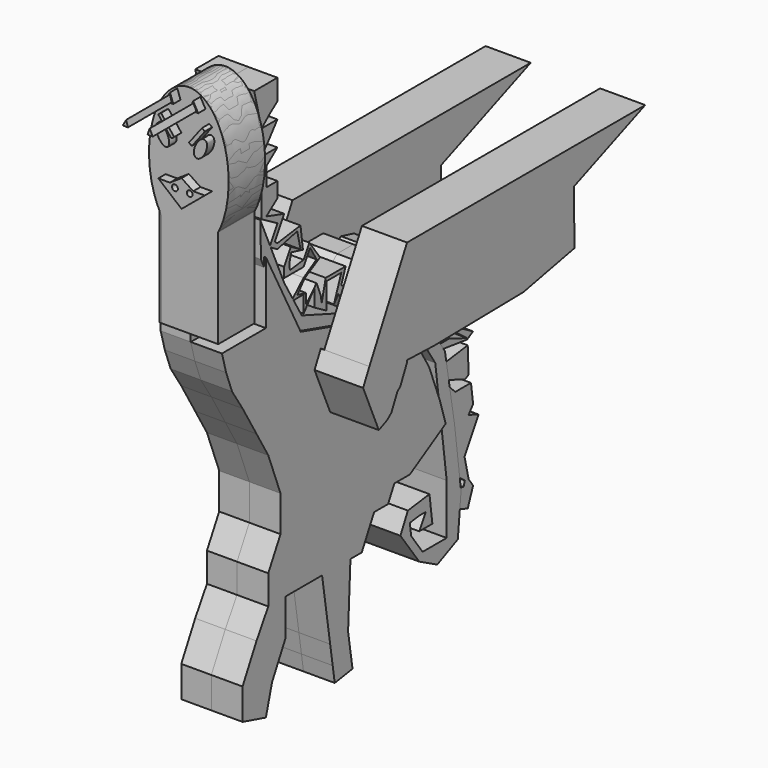
from build123d import *

# Parameters (mm, degrees)
F2_DEPTH        = 10
F3_DEPTH        = 12
F6_DEPTH        = 12
F9_DEPTH        = 6.4516
F10_DEPTH       = 6.858
F12_DEPTH       = 6.858
F11_W           = 12.0658394881
F11_H           = 1.8816260854
F13_DEPTH       = 6.604
F15_DEPTH       = 17.526
F17_DEPTH       = 9.906
F7_R            = 0.6318129406
F19_DEPTH       = 2
F20_R           = 0.6513123698
F21_DEPTH       = 2
F23_DEPTH       = 6.35
F24_DEPTH       = 6.604
F25_T1_DEPTH    = 30.4879557141
F25_T6_DEPTH    = 38.0832620454
F25_T11_DEPTH   = 30.8249260125
F25_2_T1_DEPTH  = 30.4879557141
F25_2_T6_DEPTH  = 38.0832620454
F25_2_T11_DEPTH = 30.8249260125
F27_DEPTH       = 2


# Not quite as in the source:
# - a fillet or chamfer that OpenCascade refuses, or shapes differently, is made with other operations: its cross-section is extruded or revolved along the edge and cut away or added


with BuildPart() as f2:
    # F0 (on Front) → F2 (new body)
    with BuildSketch(Plane.XZ):
        with BuildLine():
            add(Edge.make_bspline(
                [(-6.4547309206, 21.6429212113), (-3.8551533155, 16.5975436478), (0, 16.5975436478)],
                knots=[5.452422114, 5.452422114, 5.452422114, 6.2831853072, 6.2831853072, 6.2831853072], degree=2, weights=[1, 0.914962398, 1]))
            add(Edge.make_bspline(
                [(0, 16.5975436478), (3.434445083, 16.5975436478), (5.9502786025, 20.7410475478)],
                knots=[0, 0, 0, 0.7487654274, 0.7487654274, 0.7487654274], degree=2, weights=[1, 0.9307335396, 1]))
            add(Edge.make_bspline(
                [(5.9502786025, 20.7410475478), (21.313577746, 46.0439499156), (0.3582693213, 47.5674506226), (-20.5970391034, 49.0909513296), (-6.4547309206, 21.6429212113)],
                knots=[0.7487654274, 0.7487654274, 0.7487654274, 3.1005937707, 3.1005937707, 5.452422114, 5.452422114, 5.452422114], degree=2, weights=[1, 0.3846994157, 1, 0.3846994157, 1]))
        make_face()
        with BuildLine():
            add(Edge.make_bspline(
                [(0, 16.5975436478), (3.434445083, 16.5975436478), (5.9502786025, 20.7410475478)],
                knots=[0, 0, 0, 0.7487654274, 0.7487654274, 0.7487654274], degree=2, weights=[1, 0.9307335396, 1]))
            add(Edge.make_bspline(
                [(-6.4547309206, 21.6429212113), (-3.8551533155, 16.5975436478), (0, 16.5975436478)],
                knots=[5.452422114, 5.452422114, 5.452422114, 6.2831853072, 6.2831853072, 6.2831853072], degree=2, weights=[1, 0.914962398, 1]))
            Line((-6.4547309206, 21.6429212113), (-6.4547309206, 0))
            Line((-6.4547309206, 0), (5.9502786025, 0))
            Line((5.9502786025, 0), (5.9502786025, 20.7410475478))
        make_face()
    extrude(amount=F2_DEPTH)

    # F26 (on face) → F27 (join)
    with BuildSketch(Plane.XZ.offset(10)):
        with BuildLine():
            add(Edge.make_bspline(
                [(-3.1401312444, 35.7701145113), (-1.3681655429, 36.6560967536), (-3.7799722355, 39.2647554115), (-6.191778928, 41.8734140694), (-5.551937937, 38.3787731691), (-4.912096946, 34.8841322689), (-3.1401312444, 35.7701145113)],
                knots=[0, 0, 0, 2.0943951024, 2.0943951024, 4.1887902048, 4.1887902048, 6.2831853072, 6.2831853072, 6.2831853072], degree=2, weights=[1, 0.5, 1, 0.5, 1, 0.5, 1]))
        make_face()
    extrude(amount=F27_DEPTH)


with BuildPart() as f3:
    # F1 (on Front) → F3 (new body)
    with BuildSketch(Plane.XZ):
        Polygon((0, 29.1138663888), (0, 30.8139454573), (-2.5501206983, 29.1138663888), (-5.1002390683, 29.1138663888), (0, 24.8636659235), align=None)
    extrude(amount=F3_DEPTH)

    # F4: F3, F3b, F3c across plane


with BuildPart() as f3b:
    # F1 (on Front) → F3, piece 2 (new body)
    with BuildSketch(Plane.XZ):
        Polygon((-4.9794949527, 41.5934874921), (-5.0889090635, 41.4394438267), (-2.3262791801, 37.8267727792), (-2.0990670114, 37.8267727792), align=None)
        Polygon((-4.4865803793, 41.9569909573), (-4.9794949527, 41.5934874921), (-2.0990670114, 37.8267727792), (-1.6342759562, 38.227053165), align=None)
    extrude(amount=F3_DEPTH)


with BuildPart() as f3c:
    # F1 (on Front) → F3, piece 3 (new body)
    with BuildSketch(Plane.XZ):
        Polygon((-1.8204356311, 44.5381850004), (-2.5387881324, 46.5396828949), (-3.6612094846, 44.5381850004), align=None)
    extrude(amount=F3_DEPTH)


with BuildPart() as f3_1:
    add(f3.part)
    add(f3.part.mirror(Plane.YZ))
    add(f3b.part.mirror(Plane.YZ))
    add(f3c.part.mirror(Plane.YZ))

    # F7 (on face) → F19 (cut)
    with BuildSketch(Plane.XZ.offset(12)):
        with Locations((1.7824703828, 28.3940453082)):
            Circle(F7_R)
    extrude(amount=-F19_DEPTH, mode=Mode.SUBTRACT)

    # F20 (on face) → F21 (cut)
    with BuildSketch(Plane.XZ.offset(12)):
        with Locations((-1.4582620934, 28.475811705)):
            Circle(F20_R)
    extrude(amount=-F21_DEPTH, mode=Mode.SUBTRACT)


with BuildPart() as f6:
    # F5 (on face) → F6 (new body)
    with BuildSketch(Plane.XZ.offset(12)):
        Polygon((3.2756209839, 44.7876943326), (2.6005038526, 46.1258143187), (2.1202426234, 44.7876943326), align=None)
    extrude(amount=F6_DEPTH)


with BuildPart() as f6b:
    # F5 (on face) → F6, piece 2 (new body)
    with BuildSketch(Plane.XZ.offset(12)):
        Polygon((-2.162355464, 44.7876943326), (-2.5670824107, 46.1258143187), (-3.3061699942, 44.7876943326), align=None)
    extrude(amount=F6_DEPTH)


with BuildPart() as f9:
    # F8 (on Right) → F9 (new body)
    with BuildSketch(Plane.YZ):
        Polygon((8.1054354087, 4.4866758399), (1.532137394, 19.3184427917), (1.7557375602, 11.5948172129), (5.6305897209, 2.8517320687), (12.5971920788, -6.7422310822), (27.7625638992, -12.0216775686), (40.6580848693, -14.0168217382), (49.572861783, -27.8496284224), (51.4152313818, -41.9769918138), (52.6994355023, -51.8243201077), (52.6994355023, -62.9449018589), (46.0980413482, -62.9449018589), (42.9474816572, -58.6061507681), (42.596552131, -55.9152091975), (45.1674684882, -55.5799323304), (46.9695012919, -55.5799323304), (45.1674684882, -58.6061507681), (48.7715340956, -58.6061507681), (47.9822271747, -52.5537138927), (42.0558825135, -53.3265769482), (40.0054641068, -57.3544502258), (45.1674684882, -64.4632354379), (50.1269362867, -67.0540854335), (55.7603035122, -64.4632354379), (56.6465519369, -55.527344346), (54.8740550876, -41.9357679784), (52.2256828845, -26.6500413418), (42.817518115, -12.0516587049), (27.7625638992, -9.1861784458), (12.9205156118, -3.7682736292), align=None)
    extrude(amount=F9_DEPTH)

    # F8 (on Right) → F10 (join)
    with BuildSketch(Plane.YZ):
        Polygon((8.1054354087, 4.4866758399), (1.532137394, 19.3184427917), (1.7557375602, 11.5948172129), (5.6305897209, 2.8517320687), (12.5971920788, -6.7422310822), (27.7625638992, -12.0216775686), (40.6580848693, -14.0168217382), (49.572861783, -27.8496284224), (51.4152313818, -41.9769918138), (52.6994355023, -51.8243201077), (52.6994355023, -62.9449018589), (46.0980413482, -62.9449018589), (42.9474816572, -58.6061507681), (42.596552131, -55.9152091975), (45.1674684882, -55.5799323304), (46.9695012919, -55.5799323304), (45.1674684882, -58.6061507681), (48.7715340956, -58.6061507681), (47.9822271747, -52.5537138927), (42.0558825135, -53.3265769482), (40.0054641068, -57.3544502258), (45.1674684882, -64.4632354379), (50.1269362867, -67.0540854335), (55.7603035122, -64.4632354379), (56.6465519369, -55.527344346), (54.8740550876, -41.9357679784), (52.2256828845, -26.6500413418), (42.817518115, -12.0516587049), (27.7625638992, -9.1861784458), (12.9205156118, -3.7682736292), align=None)
    extrude(amount=-F10_DEPTH)

    # F11 (on Right) → F12 (join)
    with BuildSketch(Plane.YZ):
        Polygon((12.1393157169, -6.4757866785), (2.5822273456, 11.795071885), (2.5822273456, 0), (2.5822273456, -1.8816260854), (-9.4836121425, -1.8816260854), (-8.3336858079, -6.0433913022), (-6.721064914, -10.3481933475), (-3.8261981681, -14.8062761873), (0, -21.2691705674), (3.2231082692, -26.7133758606), (6.5893395804, -35.4489274323), (6.5893395804, -43.3371067047), (3.2231082692, -49.5215542614), (3.2231082692, -55.9407770634), (0, -61.2918324769), (-3.8261981681, -68.5529708862), (4.2684163239, -71.0125891538), (7.9679033037, -63.9919159361), (7.9679033037, -55.9407770634), (17.9930739105, -55.9407770634), (25.7815672235, -55.9407770634), (28.8898572326, -55.9407770634), (32.2724147794, -49.5215542614), (36.1035056412, -49.5215542614), (37.8392608134, -46.2275381138), (42.0941747725, -46.2275381138), (46.5768471874, -43.5736818115), (51.9265465413, -40.4065234666), (50.2568850148, -35.0830935564), (47.3863923786, -27.6340105488), (42.3810519278, -19.1794075072), (36.1895263195, -13.4464222938), align=None)
        Polygon((4.2684163239, -71.0125891538), (-3.8261981681, -68.5529708862), (-3.8261981681, -72.8864528992), (3.2231082692, -74.8211996529), align=None)
        Polygon((3.2231082692, -74.8211996529), (-3.8261981681, -72.8864528992), (-3.8261981681, -75.3974169493), (2.5822273456, -77.1562680602), align=None)
        Polygon((25.1365308756, -69.6748592245), (25.7815672235, -55.9407770634), (17.9930739105, -55.9407770634), (20.2164621664, -70.142770331), align=None)
        Polygon((25.7815672235, -73.795058135), (25.1365308756, -69.6748592245), (20.2164621664, -70.142770331), align=None)
        Polygon((25.7815672235, -73.795058135), (20.2164621664, -70.142770331), (20.9077002209, -74.5580847363), align=None)
        Polygon((26.3443690216, -77.3899801312), (25.7815672235, -73.795058135), (20.9077002209, -74.5580847363), (21.4705020189, -78.1530067325), align=None)
    extrude(amount=F12_DEPTH)

    # F22 (on Right) → F23 (join)
    with BuildSketch(Plane.YZ):
        Polygon((6.374317687, 21.5115565807), (2.0143464208, 19.2379765213), (6.374317687, 16.6825056076), (4.1873999871, 12.9513348546), (6.374317687, 11.6695363676), (11.8070757017, 12.9513348546), (12.7255132526, 9.0586410995), (10.064283419, 10.6184439099), (8.2402707776, 7.5064371706), (8.2402707776, 5.3265588358), (13.5636860505, 5.3265588358), (15.3341033033, 8.347124756), (17.1111002564, 5.3265588358), (13.5636860505, 3.2396173811), (10.1351579651, 0), (13.5636860505, 0), (13.5636860505, -3.7241033278), (16.5012590587, 0), (16.5012590587, -3.7241033278), (19.863597624, -5.6948407206), (19.863597624, 0), (23.9075515419, 0), (21.885574583, -5.2869431674), (23.1183427757, -3.7241033278), (25.1021422446, -7.5998823158), (30.3384047002, -2.1901051514), (34.0067259967, -2.1901051514), (30.6858606637, -5.7629146613), (30.6858606637, -9.3205478042), (38.5860130191, -4.9967369996), (42.6995791495, -4.9967369996), (40.7349355519, -7.5998823158), (36.7521606386, -8.9593110606), (36.7521606386, -11.3853020594), (41.0784259439, -14.0972314402), (43.5633193516, -7.5998823158), (48.0624114936, -9.3205478042), (48.0624114936, -11.3853020594), (44.4197580218, -12.4131189659), (43.1454405189, -14.9848153815), (52.4752251804, -14.9848153815), (54.5468328525, -18.7699061197), (49.4060702949, -16.8038355353), (45.3465212886, -19.0256562124), (48.0927578818, -24.0433798064), (51.1315829076, -22.3802087828), (54.3875972116, -23.6254625508), (58.4218000146, -26.6701526259), (53.4822099007, -24.7810198926), (48.0927578818, -24.7810198926), (50.4891980907, -29.1596209962), (50.9227966993, -29.1596209962), (50.4891980907, -25.9189717472), (58.4218000146, -26.9563752831), (60.0777398658, -26.0500673667), (56.1705380678, -23.7599741668), (55.147873642, -22.6992027075), (51.7546493685, -21.2227572942), (48.9587116034, -22.7529943547), (46.9672766634, -19.1143893965), (49.1664675286, -17.9107562517), (52.0101919188, -19.5775229623), (55.7815719124, -18.6877080364), (53.5723380744, -14.6511567863), (44.3100453781, -14.6511567863), (45.2610808354, -13.028564549), (48.8060855525, -12.1921603376), (50.4891980907, -9.3205478042), (43.5633193516, -6.3069887013), (41.0784259439, -10.5465454105), (37.872761488, -9.3205478042), (41.0784259439, -7.899916778), (43.5633193516, -4.6074424363), (40.0280356407, -3.7241033278), (31.8779945374, -7.5998823158), (32.7070372499, -5.2869431674), (35.1315699518, -1.1503698032), (30.6858606637, -1.1503698032), (26.6152015679, -4.9967369996), (23.9075515419, -2.3759328994), (25.1021422446, 0.7476106827), (19.6254998453, 0.7476106827), (18.5081807867, -3.7241033278), (18.3029319542, -2.1901051514), (17.1111002564, 0.7476106827), (14.2676095433, -2.1901051514), (14.2676095433, 0), (11.8434760085, 0.6057030017), (13.8522140785, 3.0138761345), (18.0777795613, 5.3265588358), (15.1306260624, 9.377462105), (13.5636860505, 6.7040552619), (9.805068531, 6.2011525404), (9.6304215526, 7.5064371706), (10.1351579651, 9.526484059), (13.3783222857, 8.7161349855), (12.7136140763, 13.6840618118), (6.374317687, 12.8358644653), (5.6650852585, 13.3711357547), (8.2402707776, 17.7647427445), (3.3210157141, 19.2379765213), align=None)
        Polygon((58.6017207746, -28.1321815733), (50.9227966993, -29.1596209962), (58.3676062524, -29.1596209962), (58.3676062524, -33.9571684599), (54.4010400298, -32.4401660534), (50.4891980907, -30.9440927994), (53.6639042409, -36.744684778), (58.487928737, -36.6766862571), (58.487928737, -40.385468403), (53.9383061336, -41.1653034389), (53.6639042409, -41.1653034389), (52.7907237411, -41.1653034389), (52.7907237411, -48.6471652985), (57.8177694986, -50.5697452036), (57.8177694986, -53.9344474673), (57.4758734829, -55.076067849), (57.8633627212, -55.192114329), (58.8622577488, -54.1251340254), (57.7316768195, -49.3332945378), (61.596813184, -42.7388608467), (58.8622577488, -41.6930375973), (60.0777398658, -40.0825284018), (59.4992414117, -35.7589200139), (55.147873642, -35.7589200139), (51.6759187848, -32.0609879557), (57.8940645443, -34.4391008), (58.8622577488, -33.909201622), align=None)
        Polygon((57.725328531, -48.586042255), (53.6639042409, -41.1653034389), (59.9615670733, -42.7388608467), align=None, mode=Mode.SUBTRACT)
        Polygon((50.9227966993, -29.1596209962), (50.4891980907, -29.1596209962), (50.4891980907, -30.9440927994), (54.4010400298, -32.4401660534), (58.3676062524, -33.9571684599), (58.3676062524, -29.1596209962), align=None)
        Polygon((57.2425117495, -55.8552828701), (57.4758734829, -55.076067849), (53.6639042409, -53.9344474673), (54.2127080262, -58.0361224711), (58.6017207746, -59.7146883964), (60.0777398658, -55.8552828701), (57.8633627212, -55.192114329), align=None)
        Polygon((59.9615670733, -42.7388608467), (53.6639042409, -41.1653034389), (57.725328531, -48.586042255), align=None)
        Polygon((3.3210157141, 24.8575396836), (2.0143464208, 24.8575396836), (2.0143464208, 19.2379765213), (6.374317687, 21.5115565807), (6.374317687, 24.8575396836), align=None)
        Polygon((57.8177694986, -50.5697452036), (52.7907237411, -48.6471652985), (53.6639042409, -50.7994458472), (57.8177694986, -53.9344474673), align=None)
        Polygon((58.487928737, -40.385468403), (53.6639042409, -36.744684778), (53.6639042409, -41.1653034389), (53.9383061336, -41.1653034389), align=None)
        Polygon((58.487928737, -36.6766862571), (53.6639042409, -36.744684778), (58.487928737, -40.385468403), align=None)
        Polygon((6.374317687, 31.3354618847), (2.0143464208, 31.3354618847), (2.0143464208, 27.9209110886), (3.3210157141, 28.9442409235), align=None)
        Polygon((3.3210157141, 28.9442409235), (2.0143464208, 27.9209110886), (2.0143464208, 24.8575396836), (3.3210157141, 24.8575396836), align=None)
        Polygon((58.8622577488, -54.1251340254), (57.8633627212, -55.192114329), (60.0777398658, -55.8552828701), align=None)
        Polygon((57.8633627212, -55.192114329), (57.4758734829, -55.076067849), (57.2425117495, -55.8552828701), align=None)
    extrude(amount=F23_DEPTH)


with BuildPart() as f13:
    # F11 (on Right) → F13 (new body)
    with BuildSketch(Plane.YZ):
        Polygon((12.1393157169, -6.4757866785), (2.5822273456, 11.795071885), (2.5822273456, 0), (2.5822273456, -1.8816260854), (-9.4836121425, -1.8816260854), (-8.3336858079, -6.0433913022), (-6.721064914, -10.3481933475), (-3.8261981681, -14.8062761873), (0, -21.2691705674), (3.2231082692, -26.7133758606), (6.5893395804, -35.4489274323), (6.5893395804, -43.3371067047), (3.2231082692, -49.5215542614), (3.2231082692, -55.9407770634), (0, -61.2918324769), (-3.8261981681, -68.5529708862), (4.2684163239, -71.0125891538), (7.9679033037, -63.9919159361), (7.9679033037, -55.9407770634), (17.9930739105, -55.9407770634), (25.7815672235, -55.9407770634), (28.8898572326, -55.9407770634), (32.2724147794, -49.5215542614), (36.1035056412, -49.5215542614), (37.8392608134, -46.2275381138), (42.0941747725, -46.2275381138), (46.5768471874, -43.5736818115), (51.9265465413, -40.4065234666), (50.2568850148, -35.0830935564), (47.3863923786, -27.6340105488), (42.3810519278, -19.1794075072), (36.1895263195, -13.4464222938), align=None)
        with Locations((-3.4506923985, -0.9408130427)):
            Rectangle(F11_W, F11_H)
        Polygon((25.1365308756, -69.6748592245), (25.7815672235, -55.9407770634), (17.9930739105, -55.9407770634), (20.2164621664, -70.142770331), align=None)
        Polygon((4.2684163239, -71.0125891538), (-3.8261981681, -68.5529708862), (-3.8261981681, -72.8864528992), (3.2231082692, -74.8211996529), align=None)
        Polygon((25.7815672235, -73.795058135), (25.1365308756, -69.6748592245), (20.2164621664, -70.142770331), align=None)
        Polygon((3.2231082692, -74.8211996529), (-3.8261981681, -72.8864528992), (-3.8261981681, -75.3974169493), (2.5822273456, -77.1562680602), align=None)
        Polygon((25.7815672235, -73.795058135), (20.2164621664, -70.142770331), (20.9077002209, -74.5580847363), align=None)
        Polygon((26.3443690216, -77.3899801312), (25.7815672235, -73.795058135), (20.9077002209, -74.5580847363), (21.4705020189, -78.1530067325), align=None)
    extrude(amount=-F13_DEPTH)


with BuildPart() as f15:
    # F14 (on Right) → F15 (new body)
    with BuildSketch(Plane.YZ):
        Polygon((17.6491290331, -11.953400448), (15.9272607416, -15.3971333057), (20.2319268137, -25.2978634089), (22.4355885149, -24.3397494456), (25.6127621979, -21.8541305512), (25.6127621979, -19.7017993778), (27.9803276062, -17.764698714), (27.9803276062, -14.7514333948), (25.6127621979, -14.7514333948), (22.4355885149, -14.7514333948), align=None)
    extrude(amount=F15_DEPTH)

    # F16 (on face) → F17 (join)
    with BuildSketch(Plane.YZ.offset(17.526)):
        Polygon((22.4355885149, -14.7514333948), (35.3657811751, -15.1493677909), (41.5879657357, -15.0487608429), (46.1636093004, -14.9747769342), (59.976618737, -14.7514333948), (73.9541649818, -11.953400448), (73.7608895935, 0), (93.3558419347, 7.8085386194), (27.9803276062, 7.8085386194), (17.6491290331, -11.953400448), align=None)
    extrude(amount=-F17_DEPTH)


with BuildPart() as f18_1:
    # F18: instance of F15
    add(f15.part.mirror(Plane.YZ))

    # F25#2: chamfer of 5.08 on 3 edges, made by hand

    # F25_2_s2 → F25_2_t1 (cut)
    with BuildSketch(Plane.YZ.offset(-24.0069778571)):
        Polygon((26.1171772651, -19.2890957802), (27.9803276062, -15.3573940784), (27.9803276062, -17.764698714), align=None)
    extrude(amount=F25_2_T1_DEPTH, mode=Mode.SUBTRACT)


with BuildPart() as f23:
    # F22 (on Right) → F23, piece 2 (new body)
    with BuildSketch(Plane.YZ):
        Polygon((6.374317687, 36.7647409439), (2.0143464208, 36.7647409439), (2.0143464208, 31.3354618847), (4.1873999871, 33.9406244457), align=None)
    extrude(amount=F23_DEPTH)


with BuildPart() as f23b:
    # F22 (on Right) → F23, piece 3 (new body)
    with BuildSketch(Plane.YZ):
        Polygon((6.374317687, 44.8229573667), (0, 44.8229573667), (2.0143464208, 36.7647409439), (4.1873999871, 38.6234745383), (6.374317687, 40.2723401785), (6.374317687, 42.8432300687), align=None)
    extrude(amount=F23_DEPTH)


with BuildPart() as f24:
    # F22 (on Right) → F24 (new body)
    with BuildSketch(Plane.YZ):
        Polygon((6.374317687, 21.5115565807), (2.0143464208, 19.2379765213), (6.374317687, 16.6825056076), (4.1873999871, 12.9513348546), (6.374317687, 11.6695363676), (11.8070757017, 12.9513348546), (12.7255132526, 9.0586410995), (10.064283419, 10.6184439099), (8.2402707776, 7.5064371706), (8.2402707776, 5.3265588358), (13.5636860505, 5.3265588358), (15.3341033033, 8.347124756), (17.1111002564, 5.3265588358), (13.5636860505, 3.2396173811), (10.1351579651, 0), (13.5636860505, 0), (13.5636860505, -3.7241033278), (16.5012590587, 0), (16.5012590587, -3.7241033278), (19.863597624, -5.6948407206), (19.863597624, 0), (23.9075515419, 0), (21.885574583, -5.2869431674), (23.1183427757, -3.7241033278), (25.1021422446, -7.5998823158), (30.3384047002, -2.1901051514), (34.0067259967, -2.1901051514), (30.6858606637, -5.7629146613), (30.6858606637, -9.3205478042), (38.5860130191, -4.9967369996), (42.6995791495, -4.9967369996), (40.7349355519, -7.5998823158), (36.7521606386, -8.9593110606), (36.7521606386, -11.3853020594), (41.0784259439, -14.0972314402), (43.5633193516, -7.5998823158), (48.0624114936, -9.3205478042), (48.0624114936, -11.3853020594), (44.4197580218, -12.4131189659), (43.1454405189, -14.9848153815), (52.4752251804, -14.9848153815), (54.5468328525, -18.7699061197), (49.4060702949, -16.8038355353), (45.3465212886, -19.0256562124), (48.0927578818, -24.0433798064), (51.1315829076, -22.3802087828), (54.3875972116, -23.6254625508), (58.4218000146, -26.6701526259), (53.4822099007, -24.7810198926), (48.0927578818, -24.7810198926), (50.4891980907, -29.1596209962), (50.9227966993, -29.1596209962), (50.4891980907, -25.9189717472), (58.4218000146, -26.9563752831), (60.0777398658, -26.0500673667), (56.1705380678, -23.7599741668), (55.147873642, -22.6992027075), (51.7546493685, -21.2227572942), (48.9587116034, -22.7529943547), (46.9672766634, -19.1143893965), (49.1664675286, -17.9107562517), (52.0101919188, -19.5775229623), (55.7815719124, -18.6877080364), (53.5723380744, -14.6511567863), (44.3100453781, -14.6511567863), (45.2610808354, -13.028564549), (48.8060855525, -12.1921603376), (50.4891980907, -9.3205478042), (43.5633193516, -6.3069887013), (41.0784259439, -10.5465454105), (37.872761488, -9.3205478042), (41.0784259439, -7.899916778), (43.5633193516, -4.6074424363), (40.0280356407, -3.7241033278), (31.8779945374, -7.5998823158), (32.7070372499, -5.2869431674), (35.1315699518, -1.1503698032), (30.6858606637, -1.1503698032), (26.6152015679, -4.9967369996), (23.9075515419, -2.3759328994), (25.1021422446, 0.7476106827), (19.6254998453, 0.7476106827), (18.5081807867, -3.7241033278), (18.3029319542, -2.1901051514), (17.1111002564, 0.7476106827), (14.2676095433, -2.1901051514), (14.2676095433, 0), (11.8434760085, 0.6057030017), (13.8522140785, 3.0138761345), (18.0777795613, 5.3265588358), (15.1306260624, 9.377462105), (13.5636860505, 6.7040552619), (9.805068531, 6.2011525404), (9.6304215526, 7.5064371706), (10.1351579651, 9.526484059), (13.3783222857, 8.7161349855), (12.7136140763, 13.6840618118), (6.374317687, 12.8358644653), (5.6650852585, 13.3711357547), (8.2402707776, 17.7647427445), (3.3210157141, 19.2379765213), align=None)
        Polygon((58.6017207746, -28.1321815733), (50.9227966993, -29.1596209962), (58.3676062524, -29.1596209962), (58.3676062524, -33.9571684599), (54.4010400298, -32.4401660534), (50.4891980907, -30.9440927994), (53.6639042409, -36.744684778), (58.487928737, -36.6766862571), (58.487928737, -40.385468403), (53.9383061336, -41.1653034389), (53.6639042409, -41.1653034389), (52.7907237411, -41.1653034389), (52.7907237411, -48.6471652985), (57.8177694986, -50.5697452036), (57.8177694986, -53.9344474673), (57.4758734829, -55.076067849), (57.8633627212, -55.192114329), (58.8622577488, -54.1251340254), (57.7316768195, -49.3332945378), (61.596813184, -42.7388608467), (58.8622577488, -41.6930375973), (60.0777398658, -40.0825284018), (59.4992414117, -35.7589200139), (55.147873642, -35.7589200139), (51.6759187848, -32.0609879557), (57.8940645443, -34.4391008), (58.8622577488, -33.909201622), align=None)
        Polygon((57.725328531, -48.586042255), (53.6639042409, -41.1653034389), (59.9615670733, -42.7388608467), align=None, mode=Mode.SUBTRACT)
        Polygon((50.9227966993, -29.1596209962), (50.4891980907, -29.1596209962), (50.4891980907, -30.9440927994), (54.4010400298, -32.4401660534), (58.3676062524, -33.9571684599), (58.3676062524, -29.1596209962), align=None)
        Polygon((57.2425117495, -55.8552828701), (57.4758734829, -55.076067849), (53.6639042409, -53.9344474673), (54.2127080262, -58.0361224711), (58.6017207746, -59.7146883964), (60.0777398658, -55.8552828701), (57.8633627212, -55.192114329), align=None)
        Polygon((59.9615670733, -42.7388608467), (53.6639042409, -41.1653034389), (57.725328531, -48.586042255), align=None)
        Polygon((3.3210157141, 24.8575396836), (2.0143464208, 24.8575396836), (2.0143464208, 19.2379765213), (6.374317687, 21.5115565807), (6.374317687, 24.8575396836), align=None)
        Polygon((57.8177694986, -50.5697452036), (52.7907237411, -48.6471652985), (53.6639042409, -50.7994458472), (57.8177694986, -53.9344474673), align=None)
        Polygon((58.487928737, -40.385468403), (53.6639042409, -36.744684778), (53.6639042409, -41.1653034389), (53.9383061336, -41.1653034389), align=None)
        Polygon((58.487928737, -36.6766862571), (53.6639042409, -36.744684778), (58.487928737, -40.385468403), align=None)
        Polygon((6.374317687, 31.3354618847), (2.0143464208, 31.3354618847), (2.0143464208, 27.9209110886), (3.3210157141, 28.9442409235), align=None)
        Polygon((3.3210157141, 28.9442409235), (2.0143464208, 27.9209110886), (2.0143464208, 24.8575396836), (3.3210157141, 24.8575396836), align=None)
        Polygon((58.8622577488, -54.1251340254), (57.8633627212, -55.192114329), (60.0777398658, -55.8552828701), align=None)
        Polygon((57.8633627212, -55.192114329), (57.4758734829, -55.076067849), (57.2425117495, -55.8552828701), align=None)
    extrude(amount=-F24_DEPTH)


with BuildPart() as f24b:
    # F22 (on Right) → F24, piece 2 (new body)
    with BuildSketch(Plane.YZ):
        Polygon((6.374317687, 36.7647409439), (2.0143464208, 36.7647409439), (2.0143464208, 31.3354618847), (4.1873999871, 33.9406244457), align=None)
    extrude(amount=-F24_DEPTH)


with BuildPart() as f24c:
    # F22 (on Right) → F24, piece 3 (new body)
    with BuildSketch(Plane.YZ):
        Polygon((6.374317687, 44.8229573667), (0, 44.8229573667), (2.0143464208, 36.7647409439), (4.1873999871, 38.6234745383), (6.374317687, 40.2723401785), (6.374317687, 42.8432300687), align=None)
    extrude(amount=-F24_DEPTH)


with BuildPart() as f15_1:
    add(f15.part)

    # F25: chamfer of 5.08 on 3 edges, made by hand

    # F25_s2 → F25_t1 (cut)
    with BuildSketch(Plane.YZ.offset(-6.4809778571)):
        Polygon((26.1171772651, -19.2890957802), (27.9803276062, -15.3573940784), (27.9803276062, -17.764698714), align=None)
    extrude(amount=F25_T1_DEPTH, mode=Mode.SUBTRACT)


with BuildPart() as f25_tool4:
    # F25_s5 → F25_t6 (new body)
    with BuildSketch(Plane(origin=(0, 0.4237618758, -26.2081760102), x_dir=(1, 0, 0), z_dir=(0, -0.0161669585, 0.9998693062))):
        Polygon((7.62, 68.6712495015), (12.7, 73.7512495015), (7.62, 73.7512495015), align=None)
    extrude(amount=F25_T6_DEPTH)

    split(bisect_by=Plane(origin=(0, 10.108080191, -25.3654824875), x_dir=(1, 0, 0), z_dir=(0, 0.3701870878, -0.9289572219)), keep=Keep.TOP)


with BuildPart() as f15_2:
    add(f15_1.part)

    # F25_t3: cut F25_tool4
    add(f25_tool4.part, mode=Mode.SUBTRACT)


with BuildPart() as f25_tool9:
    # F25_s10 → F25_t11 (new body)
    with BuildSketch(Plane.YZ.offset(-6.6494630063)):
        Polygon((23.6629326857, -23.3795533199), (25.6127621979, -19.3784993691), (25.6127621979, -21.8541305512), align=None)
    extrude(amount=F25_T11_DEPTH)

    split(bisect_by=Plane(origin=(0, 19.9263088451, -24.354356188), x_dir=(1, 0, 0), z_dir=(0, 0.6332381218, -0.7739570279)), keep=Keep.TOP)


with BuildPart() as f15_3:
    add(f15_2.part)

    # F25_t8: cut F25_tool9
    add(f25_tool9.part, mode=Mode.SUBTRACT)


with BuildPart() as f25_2_tool4:
    # F25_2_s5 → F25_2_t6 (new body)
    with BuildSketch(Plane(origin=(0, 0.4237618758, -26.2081760102), x_dir=(1, 0, 0), z_dir=(0, -0.0161669585, 0.9998693062))):
        Polygon((-7.62, 68.6712495015), (-12.7, 73.7512495015), (-7.62, 73.7512495015), align=None)
    extrude(amount=F25_2_T6_DEPTH)

    split(bisect_by=Plane(origin=(0, 10.108080191, -25.3654824875), x_dir=(1, 0, 0), z_dir=(0, 0.3701870878, -0.9289572219)), keep=Keep.TOP)


with BuildPart() as f18_1_1:
    add(f18_1.part)

    # F25_2_t3: cut F25_2_tool4
    add(f25_2_tool4.part, mode=Mode.SUBTRACT)


with BuildPart() as f25_2_tool9:
    # F25_2_s10 → F25_2_t11 (new body)
    with BuildSketch(Plane.YZ.offset(6.6494630063)):
        Polygon((23.6629326857, -23.3795533199), (25.6127621979, -19.3784993691), (25.6127621979, -21.8541305512), align=None)
    extrude(amount=-F25_2_T11_DEPTH)

    split(bisect_by=Plane(origin=(0, 19.9263088451, -24.354356188), x_dir=(1, 0, 0), z_dir=(0, 0.6332381218, -0.7739570279)), keep=Keep.TOP)


with BuildPart() as f18_1_2:
    add(f18_1_1.part)

    # F25_2_t8: cut F25_2_tool9
    add(f25_2_tool9.part, mode=Mode.SUBTRACT)


with BuildPart() as f28_1:
    # F28: instance of F2
    add(f2.part.mirror(Plane.YZ))


solid = Compound([f2.part, f3b.part, f3c.part, f3_1.part, f6.part, f6b.part, f9.part, f13.part, f23.part, f23b.part, f24.part, f24b.part, f24c.part, f15_3.part, f18_1_2.part, f28_1.part])
